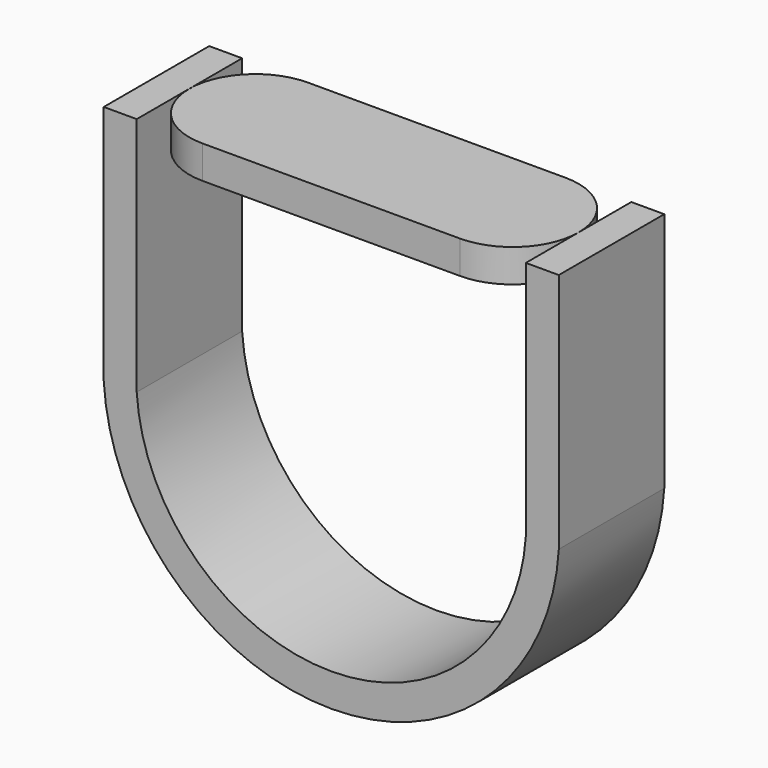
from build123d import *

# Parameters (mm, degrees)
F1_DEPTH      = 3
F1_DEPTH_BACK = 3
F2_DEPTH      = 3
F2_DEPTH_BACK = 3
F3_R          = 2.99999


# Not quite as in the source:
# - a fillet or chamfer is up to 0.001 mm smaller than in the source, because OpenCascade refuses the exact size


with BuildPart() as f1:
    # F0 (on Front) → F1 (new body, two sides)
    with BuildSketch(Plane.XZ) as f1_sk:
        with BuildLine():
            ThreePointArc((8.8570139732, -0.5647375303), (0, -8.875), (-8.8570139732, -0.5647375303))
            Line((-8.8570139732, -0.5647375303), (-8.8570139732, 8.875))
            Line((-8.8570139732, 8.875), (-8.8570139732, 10.375))
            Line((-8.8570139732, 10.375), (-10.3570139732, 10.375))
            Line((-10.3570139732, 10.375), (-10.3570139732, 8.875))
            Line((-10.3570139732, 8.875), (-10.3570139732, -0.6106443797))
            ThreePointArc((-10.3570139732, -0.6106443797), (0, -10.375), (10.3570139732, -0.6106443797))
            Line((10.3570139732, -0.6106443797), (10.3570139732, 8.875))
            Line((10.3570139732, 8.875), (10.3570139732, 10.375))
            Line((10.3570139732, 10.375), (8.8570139732, 10.375))
            Line((8.8570139732, 10.375), (8.8570139732, 8.875))
            Line((8.8570139732, 8.875), (8.8570139732, -0.5647375303))
        make_face()
    extrude(amount=F1_DEPTH)
    extrude(f1_sk.sketch, amount=-F1_DEPTH_BACK)


with BuildPart() as f2:
    # F0 (on Front) → F2 (new body, two sides)
    with BuildSketch(Plane.XZ) as f2_sk:
        Polygon((-8.8570139732, 10.375), (-8.8570139732, 8.875), (-0.6155143709, 8.875), (0.6154856291, 8.875), (8.8570139732, 8.875), (8.8570139732, 10.375), align=None)
    extrude(amount=F2_DEPTH)
    extrude(f2_sk.sketch, amount=-F2_DEPTH_BACK)

    # F3 (radius 3 in the source; OpenCascade refuses exactly that, so slightly less here)
    f3_edges = [f2.edges().sort_by_distance(p)[0] for p in [
        (-8.857014, -3, 9.625),
        (-8.857014, 3, 9.625),
        (8.857014, -3, 9.625),
        (8.857014, 3, 9.625),
    ]]
    fillet(f3_edges, radius=F3_R)


solid = Compound([f1.part, f2.part])
